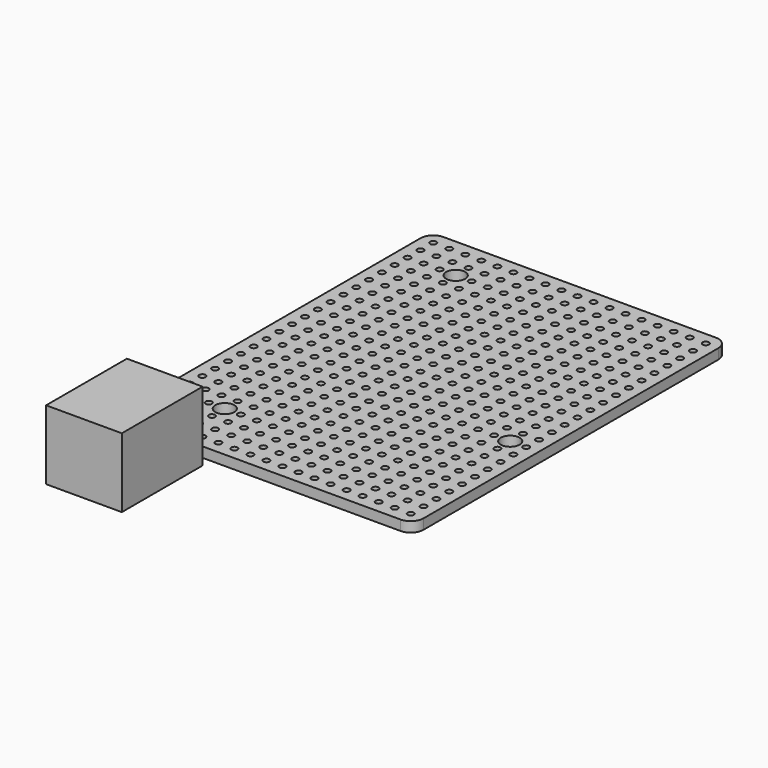
from build123d import *

# Parameters (mm, degrees)
F0_W     = 47.18
F0_H     = 62.42
F0_R     = 0.5
F0_R_2   = 1.5
F1_DEPTH = 1.6
F2_W     = 12
F2_H     = 16
F3_DEPTH = 11
F4_R     = 2


# Not quite as in the source:
# - a feature names something its author has since deleted; it is built from what else it names


with BuildPart() as f1:
    # F0 (on Top) → F1 (new body)
    with BuildSketch(Plane.XY):
        with Locations((-0.5029430622, 18.0375497397)):
            Rectangle(F0_W, F0_H)
        with Locations((-22.0929430622, -11.1724502603)):
            Circle(F0_R, mode=Mode.SUBTRACT)
        with Locations((-19.5529430622, -11.1724502603)):
            Circle(F0_R, mode=Mode.SUBTRACT)
        with Locations((-22.0929430622, -8.6324502603)):
            Circle(F0_R, mode=Mode.SUBTRACT)
        with Locations((-22.0929430622, -6.0924502603)):
            Circle(F0_R, mode=Mode.SUBTRACT)
        with Locations((-19.5529430622, -8.6324502603)):
            Circle(F0_R, mode=Mode.SUBTRACT)
        with Locations((-19.5529430622, -6.0924502603)):
            Circle(F0_R, mode=Mode.SUBTRACT)
        with Locations((-17.0129430622, -11.1724502603)):
            Circle(F0_R, mode=Mode.SUBTRACT)
        with Locations((-14.4729430622, -11.1724502603)):
            Circle(F0_R, mode=Mode.SUBTRACT)
        with Locations((-17.0129430622, -8.6324502603)):
            Circle(F0_R, mode=Mode.SUBTRACT)
        with Locations((-17.0129430622, -6.0924502603)):
            Circle(F0_R, mode=Mode.SUBTRACT)
        with Locations((-14.4729430622, -8.6324502603)):
            Circle(F0_R, mode=Mode.SUBTRACT)
        with Locations((-14.4729430622, -6.0924502603)):
            Circle(F0_R, mode=Mode.SUBTRACT)
        with Locations((-22.0929430622, -3.5524502603)):
            Circle(F0_R, mode=Mode.SUBTRACT)
        with Locations((-19.5529430622, -3.5524502603)):
            Circle(F0_R, mode=Mode.SUBTRACT)
        with Locations((-22.0929430622, -1.0124502603)):
            Circle(F0_R, mode=Mode.SUBTRACT)
        with Locations((-22.0929430622, 1.5275497397)):
            Circle(F0_R, mode=Mode.SUBTRACT)
        with Locations((-19.5529430622, -1.0124502603)):
            Circle(F0_R, mode=Mode.SUBTRACT)
        with Locations((-19.5529430622, 1.5275497397)):
            Circle(F0_R, mode=Mode.SUBTRACT)
        with Locations((-17.0129430622, -3.5524502603)):
            Circle(F0_R, mode=Mode.SUBTRACT)
        with Locations((-14.4729430622, -3.5524502603)):
            Circle(F0_R_2, mode=Mode.SUBTRACT)
        with Locations((-17.0129430622, -1.0124502603)):
            Circle(F0_R, mode=Mode.SUBTRACT)
        with Locations((-17.0129430622, 1.5275497397)):
            Circle(F0_R, mode=Mode.SUBTRACT)
        with Locations((-14.4729430622, -1.0124502603)):
            Circle(F0_R, mode=Mode.SUBTRACT)
        with Locations((-14.4729430622, 1.5275497397)):
            Circle(F0_R, mode=Mode.SUBTRACT)
        with Locations((-11.9329430622, -11.1724502603)):
            Circle(F0_R, mode=Mode.SUBTRACT)
        with Locations((-9.3929430622, -11.1724502603)):
            Circle(F0_R, mode=Mode.SUBTRACT)
        with Locations((-6.8529430622, -11.1724502603)):
            Circle(F0_R, mode=Mode.SUBTRACT)
        with Locations((-11.9329430622, -8.6324502603)):
            Circle(F0_R, mode=Mode.SUBTRACT)
        with Locations((-9.3929430622, -8.6324502603)):
            Circle(F0_R, mode=Mode.SUBTRACT)
        with Locations((-11.9329430622, -6.0924502603)):
            Circle(F0_R, mode=Mode.SUBTRACT)
        with Locations((-9.3929430622, -6.0924502603)):
            Circle(F0_R, mode=Mode.SUBTRACT)
        with Locations((-6.8529430622, -8.6324502603)):
            Circle(F0_R, mode=Mode.SUBTRACT)
        with Locations((-6.8529430622, -6.0924502603)):
            Circle(F0_R, mode=Mode.SUBTRACT)
        with Locations((-4.3129430622, -11.1724502603)):
            Circle(F0_R, mode=Mode.SUBTRACT)
        with Locations((-1.7729430622, -11.1724502603)):
            Circle(F0_R, mode=Mode.SUBTRACT)
        with Locations((-4.3129430622, -8.6324502603)):
            Circle(F0_R, mode=Mode.SUBTRACT)
        with Locations((-4.3129430622, -6.0924502603)):
            Circle(F0_R, mode=Mode.SUBTRACT)
        with Locations((-1.7729430622, -8.6324502603)):
            Circle(F0_R, mode=Mode.SUBTRACT)
        with Locations((-1.7729430622, -6.0924502603)):
            Circle(F0_R, mode=Mode.SUBTRACT)
        with Locations((-11.9329430622, -3.5524502603)):
            Circle(F0_R, mode=Mode.SUBTRACT)
        with Locations((-9.3929430622, -3.5524502603)):
            Circle(F0_R, mode=Mode.SUBTRACT)
        with Locations((-6.8529430622, -3.5524502603)):
            Circle(F0_R, mode=Mode.SUBTRACT)
        with Locations((-11.9329430622, -1.0124502603)):
            Circle(F0_R, mode=Mode.SUBTRACT)
        with Locations((-9.3929430622, -1.0124502603)):
            Circle(F0_R, mode=Mode.SUBTRACT)
        with Locations((-11.9329430622, 1.5275497397)):
            Circle(F0_R, mode=Mode.SUBTRACT)
        with Locations((-9.3929430622, 1.5275497397)):
            Circle(F0_R, mode=Mode.SUBTRACT)
        with Locations((-6.8529430622, -1.0124502603)):
            Circle(F0_R, mode=Mode.SUBTRACT)
        with Locations((-6.8529430622, 1.5275497397)):
            Circle(F0_R, mode=Mode.SUBTRACT)
        with Locations((-4.3129430622, -3.5524502603)):
            Circle(F0_R, mode=Mode.SUBTRACT)
        with Locations((-1.7729430622, -3.5524502603)):
            Circle(F0_R, mode=Mode.SUBTRACT)
        with Locations((-4.3129430622, -1.0124502603)):
            Circle(F0_R, mode=Mode.SUBTRACT)
        with Locations((-4.3129430622, 1.5275497397)):
            Circle(F0_R, mode=Mode.SUBTRACT)
        with Locations((-1.7729430622, -1.0124502603)):
            Circle(F0_R, mode=Mode.SUBTRACT)
        with Locations((-1.7729430622, 1.5275497397)):
            Circle(F0_R, mode=Mode.SUBTRACT)
        with Locations((-22.0929430622, 4.0675497397)):
            Circle(F0_R, mode=Mode.SUBTRACT)
        with Locations((-19.5529430622, 4.0675497397)):
            Circle(F0_R, mode=Mode.SUBTRACT)
        with Locations((-22.0929430622, 6.6075497397)):
            Circle(F0_R, mode=Mode.SUBTRACT)
        with Locations((-22.0929430622, 9.1475497397)):
            Circle(F0_R, mode=Mode.SUBTRACT)
        with Locations((-19.5529430622, 6.6075497397)):
            Circle(F0_R, mode=Mode.SUBTRACT)
        with Locations((-19.5529430622, 9.1475497397)):
            Circle(F0_R, mode=Mode.SUBTRACT)
        with Locations((-17.0129430622, 4.0675497397)):
            Circle(F0_R, mode=Mode.SUBTRACT)
        with Locations((-14.4729430622, 4.0675497397)):
            Circle(F0_R, mode=Mode.SUBTRACT)
        with Locations((-17.0129430622, 6.6075497397)):
            Circle(F0_R, mode=Mode.SUBTRACT)
        with Locations((-17.0129430622, 9.1475497397)):
            Circle(F0_R, mode=Mode.SUBTRACT)
        with Locations((-14.4729430622, 6.6075497397)):
            Circle(F0_R, mode=Mode.SUBTRACT)
        with Locations((-14.4729430622, 9.1475497397)):
            Circle(F0_R, mode=Mode.SUBTRACT)
        with Locations((-22.0929430622, 11.6875497397)):
            Circle(F0_R, mode=Mode.SUBTRACT)
        with Locations((-19.5529430622, 11.6875497397)):
            Circle(F0_R, mode=Mode.SUBTRACT)
        with Locations((-22.0929430622, 14.2275497397)):
            Circle(F0_R, mode=Mode.SUBTRACT)
        with Locations((-22.0929430622, 16.7675497397)):
            Circle(F0_R, mode=Mode.SUBTRACT)
        with Locations((-19.5529430622, 14.2275497397)):
            Circle(F0_R, mode=Mode.SUBTRACT)
        with Locations((-19.5529430622, 16.7675497397)):
            Circle(F0_R, mode=Mode.SUBTRACT)
        with Locations((-17.0129430622, 11.6875497397)):
            Circle(F0_R, mode=Mode.SUBTRACT)
        with Locations((-14.4729430622, 11.6875497397)):
            Circle(F0_R, mode=Mode.SUBTRACT)
        with Locations((-17.0129430622, 14.2275497397)):
            Circle(F0_R, mode=Mode.SUBTRACT)
        with Locations((-17.0129430622, 16.7675497397)):
            Circle(F0_R, mode=Mode.SUBTRACT)
        with Locations((-14.4729430622, 14.2275497397)):
            Circle(F0_R, mode=Mode.SUBTRACT)
        with Locations((-14.4729430622, 16.7675497397)):
            Circle(F0_R, mode=Mode.SUBTRACT)
        with Locations((-11.9329430622, 4.0675497397)):
            Circle(F0_R, mode=Mode.SUBTRACT)
        with Locations((-9.3929430622, 4.0675497397)):
            Circle(F0_R, mode=Mode.SUBTRACT)
        with Locations((-6.8529430622, 4.0675497397)):
            Circle(F0_R, mode=Mode.SUBTRACT)
        with Locations((-11.9329430622, 6.6075497397)):
            Circle(F0_R, mode=Mode.SUBTRACT)
        with Locations((-9.3929430622, 6.6075497397)):
            Circle(F0_R, mode=Mode.SUBTRACT)
        with Locations((-11.9329430622, 9.1475497397)):
            Circle(F0_R, mode=Mode.SUBTRACT)
        with Locations((-9.3929430622, 9.1475497397)):
            Circle(F0_R, mode=Mode.SUBTRACT)
        with Locations((-6.8529430622, 6.6075497397)):
            Circle(F0_R, mode=Mode.SUBTRACT)
        with Locations((-6.8529430622, 9.1475497397)):
            Circle(F0_R, mode=Mode.SUBTRACT)
        with Locations((-4.3129430622, 4.0675497397)):
            Circle(F0_R, mode=Mode.SUBTRACT)
        with Locations((-1.7729430622, 4.0675497397)):
            Circle(F0_R, mode=Mode.SUBTRACT)
        with Locations((-4.3129430622, 6.6075497397)):
            Circle(F0_R, mode=Mode.SUBTRACT)
        with Locations((-4.3129430622, 9.1475497397)):
            Circle(F0_R, mode=Mode.SUBTRACT)
        with Locations((-1.7729430622, 6.6075497397)):
            Circle(F0_R, mode=Mode.SUBTRACT)
        with Locations((-1.7729430622, 9.1475497397)):
            Circle(F0_R, mode=Mode.SUBTRACT)
        with Locations((-11.9329430622, 11.6875497397)):
            Circle(F0_R, mode=Mode.SUBTRACT)
        with Locations((-9.3929430622, 11.6875497397)):
            Circle(F0_R, mode=Mode.SUBTRACT)
        with Locations((-6.8529430622, 11.6875497397)):
            Circle(F0_R, mode=Mode.SUBTRACT)
        with Locations((-11.9329430622, 14.2275497397)):
            Circle(F0_R, mode=Mode.SUBTRACT)
        with Locations((-9.3929430622, 14.2275497397)):
            Circle(F0_R, mode=Mode.SUBTRACT)
        with Locations((-11.9329430622, 16.7675497397)):
            Circle(F0_R, mode=Mode.SUBTRACT)
        with Locations((-9.3929430622, 16.7675497397)):
            Circle(F0_R, mode=Mode.SUBTRACT)
        with Locations((-6.8529430622, 14.2275497397)):
            Circle(F0_R, mode=Mode.SUBTRACT)
        with Locations((-6.8529430622, 16.7675497397)):
            Circle(F0_R, mode=Mode.SUBTRACT)
        with Locations((-4.3129430622, 11.6875497397)):
            Circle(F0_R, mode=Mode.SUBTRACT)
        with Locations((-1.7729430622, 11.6875497397)):
            Circle(F0_R, mode=Mode.SUBTRACT)
        with Locations((-4.3129430622, 14.2275497397)):
            Circle(F0_R, mode=Mode.SUBTRACT)
        with Locations((-4.3129430622, 16.7675497397)):
            Circle(F0_R, mode=Mode.SUBTRACT)
        with Locations((-1.7729430622, 14.2275497397)):
            Circle(F0_R, mode=Mode.SUBTRACT)
        with Locations((-1.7729430622, 16.7675497397)):
            Circle(F0_R, mode=Mode.SUBTRACT)
        with Locations((0.7670569378, -11.1724502603)):
            Circle(F0_R, mode=Mode.SUBTRACT)
        with Locations((3.3070569378, -11.1724502603)):
            Circle(F0_R, mode=Mode.SUBTRACT)
        with Locations((0.7670569378, -8.6324502603)):
            Circle(F0_R, mode=Mode.SUBTRACT)
        with Locations((0.7670569378, -6.0924502603)):
            Circle(F0_R, mode=Mode.SUBTRACT)
        with Locations((3.3070569378, -8.6324502603)):
            Circle(F0_R, mode=Mode.SUBTRACT)
        with Locations((3.3070569378, -6.0924502603)):
            Circle(F0_R, mode=Mode.SUBTRACT)
        with Locations((5.8470569378, -11.1724502603)):
            Circle(F0_R, mode=Mode.SUBTRACT)
        with Locations((8.3870569378, -11.1724502603)):
            Circle(F0_R, mode=Mode.SUBTRACT)
        with Locations((10.9270569378, -11.1724502603)):
            Circle(F0_R, mode=Mode.SUBTRACT)
        with Locations((5.8470569378, -8.6324502603)):
            Circle(F0_R, mode=Mode.SUBTRACT)
        with Locations((5.8470569378, -6.0924502603)):
            Circle(F0_R, mode=Mode.SUBTRACT)
        with Locations((8.3870569378, -8.6324502603)):
            Circle(F0_R, mode=Mode.SUBTRACT)
        with Locations((10.9270569378, -8.6324502603)):
            Circle(F0_R, mode=Mode.SUBTRACT)
        with Locations((8.3870569378, -6.0924502603)):
            Circle(F0_R, mode=Mode.SUBTRACT)
        with Locations((10.9270569378, -6.0924502603)):
            Circle(F0_R, mode=Mode.SUBTRACT)
        with Locations((0.7670569378, -3.5524502603)):
            Circle(F0_R, mode=Mode.SUBTRACT)
        with Locations((3.3070569378, -3.5524502603)):
            Circle(F0_R, mode=Mode.SUBTRACT)
        with Locations((0.7670569378, -1.0124502603)):
            Circle(F0_R, mode=Mode.SUBTRACT)
        with Locations((0.7670569378, 1.5275497397)):
            Circle(F0_R, mode=Mode.SUBTRACT)
        with Locations((3.3070569378, -1.0124502603)):
            Circle(F0_R, mode=Mode.SUBTRACT)
        with Locations((3.3070569378, 1.5275497397)):
            Circle(F0_R, mode=Mode.SUBTRACT)
        with Locations((5.8470569378, -3.5524502603)):
            Circle(F0_R, mode=Mode.SUBTRACT)
        with Locations((8.3870569378, -3.5524502603)):
            Circle(F0_R, mode=Mode.SUBTRACT)
        with Locations((10.9270569378, -3.5524502603)):
            Circle(F0_R, mode=Mode.SUBTRACT)
        with Locations((5.8470569378, -1.0124502603)):
            Circle(F0_R, mode=Mode.SUBTRACT)
        with Locations((5.8470569378, 1.5275497397)):
            Circle(F0_R, mode=Mode.SUBTRACT)
        with Locations((8.3870569378, -1.0124502603)):
            Circle(F0_R, mode=Mode.SUBTRACT)
        with Locations((10.9270569378, -1.0124502603)):
            Circle(F0_R, mode=Mode.SUBTRACT)
        with Locations((8.3870569378, 1.5275497397)):
            Circle(F0_R, mode=Mode.SUBTRACT)
        with Locations((10.9270569378, 1.5275497397)):
            Circle(F0_R, mode=Mode.SUBTRACT)
        with Locations((13.4670569378, -11.1724502603)):
            Circle(F0_R, mode=Mode.SUBTRACT)
        with Locations((16.0070569378, -11.1724502603)):
            Circle(F0_R, mode=Mode.SUBTRACT)
        with Locations((13.4670569378, -8.6324502603)):
            Circle(F0_R, mode=Mode.SUBTRACT)
        with Locations((13.4670569378, -6.0924502603)):
            Circle(F0_R, mode=Mode.SUBTRACT)
        with Locations((16.0070569378, -8.6324502603)):
            Circle(F0_R, mode=Mode.SUBTRACT)
        with Locations((16.0070569378, -6.0924502603)):
            Circle(F0_R, mode=Mode.SUBTRACT)
        with Locations((18.5470569378, -11.1724502603)):
            Circle(F0_R, mode=Mode.SUBTRACT)
        with Locations((21.0870569378, -11.1724502603)):
            Circle(F0_R, mode=Mode.SUBTRACT)
        with Locations((18.5470569378, -8.6324502603)):
            Circle(F0_R, mode=Mode.SUBTRACT)
        with Locations((18.5470569378, -6.0924502603)):
            Circle(F0_R, mode=Mode.SUBTRACT)
        with Locations((21.0870569378, -8.6324502603)):
            Circle(F0_R, mode=Mode.SUBTRACT)
        with Locations((21.0870569378, -6.0924502603)):
            Circle(F0_R, mode=Mode.SUBTRACT)
        with Locations((13.4670569378, -3.5524502603)):
            Circle(F0_R, mode=Mode.SUBTRACT)
        with Locations((16.0070569378, -3.5524502603)):
            Circle(F0_R, mode=Mode.SUBTRACT)
        with Locations((13.4670569378, -1.0124502603)):
            Circle(F0_R, mode=Mode.SUBTRACT)
        with Locations((13.4670569378, 1.5275497397)):
            Circle(F0_R, mode=Mode.SUBTRACT)
        with Locations((16.0070569378, -1.0124502603)):
            Circle(F0_R, mode=Mode.SUBTRACT)
        with Locations((16.0070569378, 1.5275497397)):
            Circle(F0_R, mode=Mode.SUBTRACT)
        with Locations((18.5470569378, -3.5524502603)):
            Circle(F0_R, mode=Mode.SUBTRACT)
        with Locations((21.0870569378, -3.5524502603)):
            Circle(F0_R, mode=Mode.SUBTRACT)
        with Locations((18.5470569378, -1.0124502603)):
            Circle(F0_R, mode=Mode.SUBTRACT)
        with Locations((18.5470569378, 1.5275497397)):
            Circle(F0_R, mode=Mode.SUBTRACT)
        with Locations((21.0870569378, -1.0124502603)):
            Circle(F0_R, mode=Mode.SUBTRACT)
        with Locations((21.0870569378, 1.5275497397)):
            Circle(F0_R, mode=Mode.SUBTRACT)
        with Locations((0.7670569378, 4.0675497397)):
            Circle(F0_R, mode=Mode.SUBTRACT)
        with Locations((3.3070569378, 4.0675497397)):
            Circle(F0_R, mode=Mode.SUBTRACT)
        with Locations((0.7670569378, 6.6075497397)):
            Circle(F0_R, mode=Mode.SUBTRACT)
        with Locations((0.7670569378, 9.1475497397)):
            Circle(F0_R, mode=Mode.SUBTRACT)
        with Locations((3.3070569378, 6.6075497397)):
            Circle(F0_R, mode=Mode.SUBTRACT)
        with Locations((3.3070569378, 9.1475497397)):
            Circle(F0_R, mode=Mode.SUBTRACT)
        with Locations((5.8470569378, 4.0675497397)):
            Circle(F0_R, mode=Mode.SUBTRACT)
        with Locations((8.3870569378, 4.0675497397)):
            Circle(F0_R, mode=Mode.SUBTRACT)
        with Locations((10.9270569378, 4.0675497397)):
            Circle(F0_R, mode=Mode.SUBTRACT)
        with Locations((5.8470569378, 6.6075497397)):
            Circle(F0_R, mode=Mode.SUBTRACT)
        with Locations((5.8470569378, 9.1475497397)):
            Circle(F0_R, mode=Mode.SUBTRACT)
        with Locations((8.3870569378, 6.6075497397)):
            Circle(F0_R, mode=Mode.SUBTRACT)
        with Locations((10.9270569378, 6.6075497397)):
            Circle(F0_R, mode=Mode.SUBTRACT)
        with Locations((8.3870569378, 9.1475497397)):
            Circle(F0_R, mode=Mode.SUBTRACT)
        with Locations((10.9270569378, 9.1475497397)):
            Circle(F0_R, mode=Mode.SUBTRACT)
        with Locations((0.7670569378, 11.6875497397)):
            Circle(F0_R, mode=Mode.SUBTRACT)
        with Locations((3.3070569378, 11.6875497397)):
            Circle(F0_R, mode=Mode.SUBTRACT)
        with Locations((0.7670569378, 14.2275497397)):
            Circle(F0_R, mode=Mode.SUBTRACT)
        with Locations((0.7670569378, 16.7675497397)):
            Circle(F0_R, mode=Mode.SUBTRACT)
        with Locations((3.3070569378, 14.2275497397)):
            Circle(F0_R, mode=Mode.SUBTRACT)
        with Locations((3.3070569378, 16.7675497397)):
            Circle(F0_R, mode=Mode.SUBTRACT)
        with Locations((5.8470569378, 11.6875497397)):
            Circle(F0_R, mode=Mode.SUBTRACT)
        with Locations((8.3870569378, 11.6875497397)):
            Circle(F0_R, mode=Mode.SUBTRACT)
        with Locations((10.9270569378, 11.6875497397)):
            Circle(F0_R, mode=Mode.SUBTRACT)
        with Locations((5.8470569378, 14.2275497397)):
            Circle(F0_R, mode=Mode.SUBTRACT)
        with Locations((5.8470569378, 16.7675497397)):
            Circle(F0_R, mode=Mode.SUBTRACT)
        with Locations((8.3870569378, 14.2275497397)):
            Circle(F0_R, mode=Mode.SUBTRACT)
        with Locations((10.9270569378, 14.2275497397)):
            Circle(F0_R, mode=Mode.SUBTRACT)
        with Locations((8.3870569378, 16.7675497397)):
            Circle(F0_R, mode=Mode.SUBTRACT)
        with Locations((10.9270569378, 16.7675497397)):
            Circle(F0_R, mode=Mode.SUBTRACT)
        with Locations((13.4670569378, 4.0675497397)):
            Circle(F0_R, mode=Mode.SUBTRACT)
        with Locations((16.0070569378, 4.0675497397)):
            Circle(F0_R, mode=Mode.SUBTRACT)
        with Locations((13.4670569378, 6.6075497397)):
            Circle(F0_R, mode=Mode.SUBTRACT)
        with Locations((13.4670569378, 9.1475497397)):
            Circle(F0_R, mode=Mode.SUBTRACT)
        with Locations((16.0070569378, 6.6075497397)):
            Circle(F0_R, mode=Mode.SUBTRACT)
        with Locations((16.0070569378, 9.1475497397)):
            Circle(F0_R, mode=Mode.SUBTRACT)
        with Locations((18.5470569378, 4.0675497397)):
            Circle(F0_R, mode=Mode.SUBTRACT)
        with Locations((21.0870569378, 4.0675497397)):
            Circle(F0_R, mode=Mode.SUBTRACT)
        with Locations((18.5470569378, 6.6075497397)):
            Circle(F0_R, mode=Mode.SUBTRACT)
        with Locations((18.5470569378, 9.1475497397)):
            Circle(F0_R, mode=Mode.SUBTRACT)
        with Locations((21.0870569378, 6.6075497397)):
            Circle(F0_R, mode=Mode.SUBTRACT)
        with Locations((21.0870569378, 9.1475497397)):
            Circle(F0_R, mode=Mode.SUBTRACT)
        with Locations((13.4670569378, 11.6875497397)):
            Circle(F0_R, mode=Mode.SUBTRACT)
        with Locations((16.0070569378, 11.6875497397)):
            Circle(F0_R, mode=Mode.SUBTRACT)
        with Locations((13.4670569378, 14.2275497397)):
            Circle(F0_R, mode=Mode.SUBTRACT)
        with Locations((13.4670569378, 16.7675497397)):
            Circle(F0_R, mode=Mode.SUBTRACT)
        with Locations((16.0070569378, 14.2275497397)):
            Circle(F0_R, mode=Mode.SUBTRACT)
        with Locations((16.0070569378, 16.7675497397)):
            Circle(F0_R, mode=Mode.SUBTRACT)
        with Locations((18.5470569378, 11.6875497397)):
            Circle(F0_R_2, mode=Mode.SUBTRACT)
        with Locations((21.0870569378, 11.6875497397)):
            Circle(F0_R, mode=Mode.SUBTRACT)
        with Locations((18.5470569378, 14.2275497397)):
            Circle(F0_R, mode=Mode.SUBTRACT)
        with Locations((18.5470569378, 16.7675497397)):
            Circle(F0_R, mode=Mode.SUBTRACT)
        with Locations((21.0870569378, 14.2275497397)):
            Circle(F0_R, mode=Mode.SUBTRACT)
        with Locations((21.0870569378, 16.7675497397)):
            Circle(F0_R, mode=Mode.SUBTRACT)
        with Locations((-22.0929430622, 19.3075497397)):
            Circle(F0_R, mode=Mode.SUBTRACT)
        with Locations((-22.0929430622, 21.8475497397)):
            Circle(F0_R, mode=Mode.SUBTRACT)
        with Locations((-19.5529430622, 19.3075497397)):
            Circle(F0_R, mode=Mode.SUBTRACT)
        with Locations((-19.5529430622, 21.8475497397)):
            Circle(F0_R, mode=Mode.SUBTRACT)
        with Locations((-22.0929430622, 24.3875497397)):
            Circle(F0_R, mode=Mode.SUBTRACT)
        with Locations((-19.5529430622, 24.3875497397)):
            Circle(F0_R, mode=Mode.SUBTRACT)
        with Locations((-17.0129430622, 19.3075497397)):
            Circle(F0_R, mode=Mode.SUBTRACT)
        with Locations((-17.0129430622, 21.8475497397)):
            Circle(F0_R, mode=Mode.SUBTRACT)
        with Locations((-14.4729430622, 19.3075497397)):
            Circle(F0_R, mode=Mode.SUBTRACT)
        with Locations((-14.4729430622, 21.8475497397)):
            Circle(F0_R, mode=Mode.SUBTRACT)
        with Locations((-17.0129430622, 24.3875497397)):
            Circle(F0_R, mode=Mode.SUBTRACT)
        with Locations((-14.4729430622, 24.3875497397)):
            Circle(F0_R, mode=Mode.SUBTRACT)
        with Locations((-22.0929430622, 26.9275497397)):
            Circle(F0_R, mode=Mode.SUBTRACT)
        with Locations((-22.0929430622, 29.4675497397)):
            Circle(F0_R, mode=Mode.SUBTRACT)
        with Locations((-19.5529430622, 26.9275497397)):
            Circle(F0_R, mode=Mode.SUBTRACT)
        with Locations((-19.5529430622, 29.4675497397)):
            Circle(F0_R, mode=Mode.SUBTRACT)
        with Locations((-22.0929430622, 32.0075497397)):
            Circle(F0_R, mode=Mode.SUBTRACT)
        with Locations((-19.5529430622, 32.0075497397)):
            Circle(F0_R, mode=Mode.SUBTRACT)
        with Locations((-17.0129430622, 26.9275497397)):
            Circle(F0_R, mode=Mode.SUBTRACT)
        with Locations((-17.0129430622, 29.4675497397)):
            Circle(F0_R, mode=Mode.SUBTRACT)
        with Locations((-14.4729430622, 26.9275497397)):
            Circle(F0_R, mode=Mode.SUBTRACT)
        with Locations((-14.4729430622, 29.4675497397)):
            Circle(F0_R, mode=Mode.SUBTRACT)
        with Locations((-17.0129430622, 32.0075497397)):
            Circle(F0_R, mode=Mode.SUBTRACT)
        with Locations((-14.4729430622, 32.0075497397)):
            Circle(F0_R, mode=Mode.SUBTRACT)
        with Locations((-11.9329430622, 19.3075497397)):
            Circle(F0_R, mode=Mode.SUBTRACT)
        with Locations((-9.3929430622, 19.3075497397)):
            Circle(F0_R, mode=Mode.SUBTRACT)
        with Locations((-11.9329430622, 21.8475497397)):
            Circle(F0_R, mode=Mode.SUBTRACT)
        with Locations((-9.3929430622, 21.8475497397)):
            Circle(F0_R, mode=Mode.SUBTRACT)
        with Locations((-6.8529430622, 19.3075497397)):
            Circle(F0_R, mode=Mode.SUBTRACT)
        with Locations((-6.8529430622, 21.8475497397)):
            Circle(F0_R, mode=Mode.SUBTRACT)
        with Locations((-11.9329430622, 24.3875497397)):
            Circle(F0_R, mode=Mode.SUBTRACT)
        with Locations((-9.3929430622, 24.3875497397)):
            Circle(F0_R, mode=Mode.SUBTRACT)
        with Locations((-6.8529430622, 24.3875497397)):
            Circle(F0_R, mode=Mode.SUBTRACT)
        with Locations((-4.3129430622, 19.3075497397)):
            Circle(F0_R, mode=Mode.SUBTRACT)
        with Locations((-4.3129430622, 21.8475497397)):
            Circle(F0_R, mode=Mode.SUBTRACT)
        with Locations((-1.7729430622, 19.3075497397)):
            Circle(F0_R, mode=Mode.SUBTRACT)
        with Locations((-1.7729430622, 21.8475497397)):
            Circle(F0_R, mode=Mode.SUBTRACT)
        with Locations((-4.3129430622, 24.3875497397)):
            Circle(F0_R, mode=Mode.SUBTRACT)
        with Locations((-1.7729430622, 24.3875497397)):
            Circle(F0_R, mode=Mode.SUBTRACT)
        with Locations((-11.9329430622, 26.9275497397)):
            Circle(F0_R, mode=Mode.SUBTRACT)
        with Locations((-9.3929430622, 26.9275497397)):
            Circle(F0_R, mode=Mode.SUBTRACT)
        with Locations((-11.9329430622, 29.4675497397)):
            Circle(F0_R, mode=Mode.SUBTRACT)
        with Locations((-9.3929430622, 29.4675497397)):
            Circle(F0_R, mode=Mode.SUBTRACT)
        with Locations((-6.8529430622, 26.9275497397)):
            Circle(F0_R, mode=Mode.SUBTRACT)
        with Locations((-6.8529430622, 29.4675497397)):
            Circle(F0_R, mode=Mode.SUBTRACT)
        with Locations((-11.9329430622, 32.0075497397)):
            Circle(F0_R, mode=Mode.SUBTRACT)
        with Locations((-9.3929430622, 32.0075497397)):
            Circle(F0_R, mode=Mode.SUBTRACT)
        with Locations((-6.8529430622, 32.0075497397)):
            Circle(F0_R, mode=Mode.SUBTRACT)
        with Locations((-4.3129430622, 26.9275497397)):
            Circle(F0_R, mode=Mode.SUBTRACT)
        with Locations((-4.3129430622, 29.4675497397)):
            Circle(F0_R, mode=Mode.SUBTRACT)
        with Locations((-1.7729430622, 26.9275497397)):
            Circle(F0_R, mode=Mode.SUBTRACT)
        with Locations((-1.7729430622, 29.4675497397)):
            Circle(F0_R, mode=Mode.SUBTRACT)
        with Locations((-4.3129430622, 32.0075497397)):
            Circle(F0_R, mode=Mode.SUBTRACT)
        with Locations((-1.7729430622, 32.0075497397)):
            Circle(F0_R, mode=Mode.SUBTRACT)
        with Locations((-22.0929430622, 34.5475497397)):
            Circle(F0_R, mode=Mode.SUBTRACT)
        with Locations((-22.0929430622, 37.0875497397)):
            Circle(F0_R, mode=Mode.SUBTRACT)
        with Locations((-19.5529430622, 34.5475497397)):
            Circle(F0_R, mode=Mode.SUBTRACT)
        with Locations((-19.5529430622, 37.0875497397)):
            Circle(F0_R, mode=Mode.SUBTRACT)
        with Locations((-22.0929430622, 39.6275497397)):
            Circle(F0_R, mode=Mode.SUBTRACT)
        with Locations((-19.5529430622, 39.6275497397)):
            Circle(F0_R, mode=Mode.SUBTRACT)
        with Locations((-17.0129430622, 34.5475497397)):
            Circle(F0_R, mode=Mode.SUBTRACT)
        with Locations((-17.0129430622, 37.0875497397)):
            Circle(F0_R, mode=Mode.SUBTRACT)
        with Locations((-14.4729430622, 34.5475497397)):
            Circle(F0_R, mode=Mode.SUBTRACT)
        with Locations((-14.4729430622, 37.0875497397)):
            Circle(F0_R, mode=Mode.SUBTRACT)
        with Locations((-17.0129430622, 39.6275497397)):
            Circle(F0_R, mode=Mode.SUBTRACT)
        with Locations((-14.4729430622, 39.6275497397)):
            Circle(F0_R, mode=Mode.SUBTRACT)
        with Locations((-22.0929430622, 42.1675497397)):
            Circle(F0_R, mode=Mode.SUBTRACT)
        with Locations((-22.0929430622, 44.7075497397)):
            Circle(F0_R, mode=Mode.SUBTRACT)
        with Locations((-19.5529430622, 42.1675497397)):
            Circle(F0_R, mode=Mode.SUBTRACT)
        with Locations((-19.5529430622, 44.7075497397)):
            Circle(F0_R, mode=Mode.SUBTRACT)
        with Locations((-22.0929430622, 47.2475497397)):
            Circle(F0_R, mode=Mode.SUBTRACT)
        with Locations((-19.5529430622, 47.2475497397)):
            Circle(F0_R, mode=Mode.SUBTRACT)
        with Locations((-17.0129430622, 42.1675497397)):
            Circle(F0_R, mode=Mode.SUBTRACT)
        with Locations((-17.0129430622, 44.7075497397)):
            Circle(F0_R, mode=Mode.SUBTRACT)
        with Locations((-14.4729430622, 42.1675497397)):
            Circle(F0_R_2, mode=Mode.SUBTRACT)
        with Locations((-14.4729430622, 44.7075497397)):
            Circle(F0_R, mode=Mode.SUBTRACT)
        with Locations((-17.0129430622, 47.2475497397)):
            Circle(F0_R, mode=Mode.SUBTRACT)
        with Locations((-14.4729430622, 47.2475497397)):
            Circle(F0_R, mode=Mode.SUBTRACT)
        with Locations((-11.9329430622, 34.5475497397)):
            Circle(F0_R, mode=Mode.SUBTRACT)
        with Locations((-9.3929430622, 34.5475497397)):
            Circle(F0_R, mode=Mode.SUBTRACT)
        with Locations((-11.9329430622, 37.0875497397)):
            Circle(F0_R, mode=Mode.SUBTRACT)
        with Locations((-9.3929430622, 37.0875497397)):
            Circle(F0_R, mode=Mode.SUBTRACT)
        with Locations((-6.8529430622, 34.5475497397)):
            Circle(F0_R, mode=Mode.SUBTRACT)
        with Locations((-6.8529430622, 37.0875497397)):
            Circle(F0_R, mode=Mode.SUBTRACT)
        with Locations((-11.9329430622, 39.6275497397)):
            Circle(F0_R, mode=Mode.SUBTRACT)
        with Locations((-9.3929430622, 39.6275497397)):
            Circle(F0_R, mode=Mode.SUBTRACT)
        with Locations((-6.8529430622, 39.6275497397)):
            Circle(F0_R, mode=Mode.SUBTRACT)
        with Locations((-4.3129430622, 34.5475497397)):
            Circle(F0_R, mode=Mode.SUBTRACT)
        with Locations((-4.3129430622, 37.0875497397)):
            Circle(F0_R, mode=Mode.SUBTRACT)
        with Locations((-1.7729430622, 34.5475497397)):
            Circle(F0_R, mode=Mode.SUBTRACT)
        with Locations((-1.7729430622, 37.0875497397)):
            Circle(F0_R, mode=Mode.SUBTRACT)
        with Locations((-4.3129430622, 39.6275497397)):
            Circle(F0_R, mode=Mode.SUBTRACT)
        with Locations((-1.7729430622, 39.6275497397)):
            Circle(F0_R, mode=Mode.SUBTRACT)
        with Locations((-11.9329430622, 42.1675497397)):
            Circle(F0_R, mode=Mode.SUBTRACT)
        with Locations((-9.3929430622, 42.1675497397)):
            Circle(F0_R, mode=Mode.SUBTRACT)
        with Locations((-11.9329430622, 44.7075497397)):
            Circle(F0_R, mode=Mode.SUBTRACT)
        with Locations((-9.3929430622, 44.7075497397)):
            Circle(F0_R, mode=Mode.SUBTRACT)
        with Locations((-6.8529430622, 42.1675497397)):
            Circle(F0_R, mode=Mode.SUBTRACT)
        with Locations((-6.8529430622, 44.7075497397)):
            Circle(F0_R, mode=Mode.SUBTRACT)
        with Locations((-11.9329430622, 47.2475497397)):
            Circle(F0_R, mode=Mode.SUBTRACT)
        with Locations((-9.3929430622, 47.2475497397)):
            Circle(F0_R, mode=Mode.SUBTRACT)
        with Locations((-6.8529430622, 47.2475497397)):
            Circle(F0_R, mode=Mode.SUBTRACT)
        with Locations((-4.3129430622, 42.1675497397)):
            Circle(F0_R, mode=Mode.SUBTRACT)
        with Locations((-4.3129430622, 44.7075497397)):
            Circle(F0_R, mode=Mode.SUBTRACT)
        with Locations((-1.7729430622, 42.1675497397)):
            Circle(F0_R, mode=Mode.SUBTRACT)
        with Locations((-1.7729430622, 44.7075497397)):
            Circle(F0_R, mode=Mode.SUBTRACT)
        with Locations((-4.3129430622, 47.2475497397)):
            Circle(F0_R, mode=Mode.SUBTRACT)
        with Locations((-1.7729430622, 47.2475497397)):
            Circle(F0_R, mode=Mode.SUBTRACT)
        with Locations((0.7670569378, 19.3075497397)):
            Circle(F0_R, mode=Mode.SUBTRACT)
        with Locations((0.7670569378, 21.8475497397)):
            Circle(F0_R, mode=Mode.SUBTRACT)
        with Locations((3.3070569378, 19.3075497397)):
            Circle(F0_R, mode=Mode.SUBTRACT)
        with Locations((3.3070569378, 21.8475497397)):
            Circle(F0_R, mode=Mode.SUBTRACT)
        with Locations((0.7670569378, 24.3875497397)):
            Circle(F0_R, mode=Mode.SUBTRACT)
        with Locations((3.3070569378, 24.3875497397)):
            Circle(F0_R, mode=Mode.SUBTRACT)
        with Locations((5.8470569378, 19.3075497397)):
            Circle(F0_R, mode=Mode.SUBTRACT)
        with Locations((5.8470569378, 21.8475497397)):
            Circle(F0_R, mode=Mode.SUBTRACT)
        with Locations((8.3870569378, 19.3075497397)):
            Circle(F0_R, mode=Mode.SUBTRACT)
        with Locations((10.9270569378, 19.3075497397)):
            Circle(F0_R, mode=Mode.SUBTRACT)
        with Locations((8.3870569378, 21.8475497397)):
            Circle(F0_R, mode=Mode.SUBTRACT)
        with Locations((10.9270569378, 21.8475497397)):
            Circle(F0_R, mode=Mode.SUBTRACT)
        with Locations((5.8470569378, 24.3875497397)):
            Circle(F0_R, mode=Mode.SUBTRACT)
        with Locations((8.3870569378, 24.3875497397)):
            Circle(F0_R, mode=Mode.SUBTRACT)
        with Locations((10.9270569378, 24.3875497397)):
            Circle(F0_R, mode=Mode.SUBTRACT)
        with Locations((0.7670569378, 26.9275497397)):
            Circle(F0_R, mode=Mode.SUBTRACT)
        with Locations((0.7670569378, 29.4675497397)):
            Circle(F0_R, mode=Mode.SUBTRACT)
        with Locations((3.3070569378, 26.9275497397)):
            Circle(F0_R, mode=Mode.SUBTRACT)
        with Locations((3.3070569378, 29.4675497397)):
            Circle(F0_R, mode=Mode.SUBTRACT)
        with Locations((0.7670569378, 32.0075497397)):
            Circle(F0_R, mode=Mode.SUBTRACT)
        with Locations((3.3070569378, 32.0075497397)):
            Circle(F0_R, mode=Mode.SUBTRACT)
        with Locations((5.8470569378, 26.9275497397)):
            Circle(F0_R, mode=Mode.SUBTRACT)
        with Locations((5.8470569378, 29.4675497397)):
            Circle(F0_R, mode=Mode.SUBTRACT)
        with Locations((8.3870569378, 26.9275497397)):
            Circle(F0_R, mode=Mode.SUBTRACT)
        with Locations((10.9270569378, 26.9275497397)):
            Circle(F0_R, mode=Mode.SUBTRACT)
        with Locations((8.3870569378, 29.4675497397)):
            Circle(F0_R, mode=Mode.SUBTRACT)
        with Locations((10.9270569378, 29.4675497397)):
            Circle(F0_R, mode=Mode.SUBTRACT)
        with Locations((5.8470569378, 32.0075497397)):
            Circle(F0_R, mode=Mode.SUBTRACT)
        with Locations((8.3870569378, 32.0075497397)):
            Circle(F0_R, mode=Mode.SUBTRACT)
        with Locations((10.9270569378, 32.0075497397)):
            Circle(F0_R, mode=Mode.SUBTRACT)
        with Locations((13.4670569378, 19.3075497397)):
            Circle(F0_R, mode=Mode.SUBTRACT)
        with Locations((13.4670569378, 21.8475497397)):
            Circle(F0_R, mode=Mode.SUBTRACT)
        with Locations((16.0070569378, 19.3075497397)):
            Circle(F0_R, mode=Mode.SUBTRACT)
        with Locations((16.0070569378, 21.8475497397)):
            Circle(F0_R, mode=Mode.SUBTRACT)
        with Locations((13.4670569378, 24.3875497397)):
            Circle(F0_R, mode=Mode.SUBTRACT)
        with Locations((16.0070569378, 24.3875497397)):
            Circle(F0_R, mode=Mode.SUBTRACT)
        with Locations((18.5470569378, 19.3075497397)):
            Circle(F0_R, mode=Mode.SUBTRACT)
        with Locations((18.5470569378, 21.8475497397)):
            Circle(F0_R, mode=Mode.SUBTRACT)
        with Locations((21.0870569378, 19.3075497397)):
            Circle(F0_R, mode=Mode.SUBTRACT)
        with Locations((21.0870569378, 21.8475497397)):
            Circle(F0_R, mode=Mode.SUBTRACT)
        with Locations((18.5470569378, 24.3875497397)):
            Circle(F0_R, mode=Mode.SUBTRACT)
        with Locations((21.0870569378, 24.3875497397)):
            Circle(F0_R, mode=Mode.SUBTRACT)
        with Locations((13.4670569378, 26.9275497397)):
            Circle(F0_R, mode=Mode.SUBTRACT)
        with Locations((13.4670569378, 29.4675497397)):
            Circle(F0_R, mode=Mode.SUBTRACT)
        with Locations((16.0070569378, 26.9275497397)):
            Circle(F0_R, mode=Mode.SUBTRACT)
        with Locations((16.0070569378, 29.4675497397)):
            Circle(F0_R, mode=Mode.SUBTRACT)
        with Locations((13.4670569378, 32.0075497397)):
            Circle(F0_R, mode=Mode.SUBTRACT)
        with Locations((16.0070569378, 32.0075497397)):
            Circle(F0_R, mode=Mode.SUBTRACT)
        with Locations((18.5470569378, 26.9275497397)):
            Circle(F0_R, mode=Mode.SUBTRACT)
        with Locations((18.5470569378, 29.4675497397)):
            Circle(F0_R, mode=Mode.SUBTRACT)
        with Locations((21.0870569378, 26.9275497397)):
            Circle(F0_R, mode=Mode.SUBTRACT)
        with Locations((21.0870569378, 29.4675497397)):
            Circle(F0_R, mode=Mode.SUBTRACT)
        with Locations((18.5470569378, 32.0075497397)):
            Circle(F0_R, mode=Mode.SUBTRACT)
        with Locations((21.0870569378, 32.0075497397)):
            Circle(F0_R, mode=Mode.SUBTRACT)
        with Locations((0.7670569378, 34.5475497397)):
            Circle(F0_R, mode=Mode.SUBTRACT)
        with Locations((0.7670569378, 37.0875497397)):
            Circle(F0_R, mode=Mode.SUBTRACT)
        with Locations((3.3070569378, 34.5475497397)):
            Circle(F0_R, mode=Mode.SUBTRACT)
        with Locations((3.3070569378, 37.0875497397)):
            Circle(F0_R, mode=Mode.SUBTRACT)
        with Locations((0.7670569378, 39.6275497397)):
            Circle(F0_R, mode=Mode.SUBTRACT)
        with Locations((3.3070569378, 39.6275497397)):
            Circle(F0_R, mode=Mode.SUBTRACT)
        with Locations((5.8470569378, 34.5475497397)):
            Circle(F0_R, mode=Mode.SUBTRACT)
        with Locations((5.8470569378, 37.0875497397)):
            Circle(F0_R, mode=Mode.SUBTRACT)
        with Locations((8.3870569378, 34.5475497397)):
            Circle(F0_R, mode=Mode.SUBTRACT)
        with Locations((10.9270569378, 34.5475497397)):
            Circle(F0_R, mode=Mode.SUBTRACT)
        with Locations((8.3870569378, 37.0875497397)):
            Circle(F0_R, mode=Mode.SUBTRACT)
        with Locations((10.9270569378, 37.0875497397)):
            Circle(F0_R, mode=Mode.SUBTRACT)
        with Locations((5.8470569378, 39.6275497397)):
            Circle(F0_R, mode=Mode.SUBTRACT)
        with Locations((8.3870569378, 39.6275497397)):
            Circle(F0_R, mode=Mode.SUBTRACT)
        with Locations((10.9270569378, 39.6275497397)):
            Circle(F0_R, mode=Mode.SUBTRACT)
        with Locations((0.7670569378, 42.1675497397)):
            Circle(F0_R, mode=Mode.SUBTRACT)
        with Locations((0.7670569378, 44.7075497397)):
            Circle(F0_R, mode=Mode.SUBTRACT)
        with Locations((3.3070569378, 42.1675497397)):
            Circle(F0_R, mode=Mode.SUBTRACT)
        with Locations((3.3070569378, 44.7075497397)):
            Circle(F0_R, mode=Mode.SUBTRACT)
        with Locations((0.7670569378, 47.2475497397)):
            Circle(F0_R, mode=Mode.SUBTRACT)
        with Locations((3.3070569378, 47.2475497397)):
            Circle(F0_R, mode=Mode.SUBTRACT)
        with Locations((5.8470569378, 42.1675497397)):
            Circle(F0_R, mode=Mode.SUBTRACT)
        with Locations((5.8470569378, 44.7075497397)):
            Circle(F0_R, mode=Mode.SUBTRACT)
        with Locations((8.3870569378, 42.1675497397)):
            Circle(F0_R, mode=Mode.SUBTRACT)
        with Locations((10.9270569378, 42.1675497397)):
            Circle(F0_R, mode=Mode.SUBTRACT)
        with Locations((8.3870569378, 44.7075497397)):
            Circle(F0_R, mode=Mode.SUBTRACT)
        with Locations((10.9270569378, 44.7075497397)):
            Circle(F0_R, mode=Mode.SUBTRACT)
        with Locations((5.8470569378, 47.2475497397)):
            Circle(F0_R, mode=Mode.SUBTRACT)
        with Locations((8.3870569378, 47.2475497397)):
            Circle(F0_R, mode=Mode.SUBTRACT)
        with Locations((10.9270569378, 47.2475497397)):
            Circle(F0_R, mode=Mode.SUBTRACT)
        with Locations((13.4670569378, 34.5475497397)):
            Circle(F0_R, mode=Mode.SUBTRACT)
        with Locations((13.4670569378, 37.0875497397)):
            Circle(F0_R, mode=Mode.SUBTRACT)
        with Locations((16.0070569378, 34.5475497397)):
            Circle(F0_R, mode=Mode.SUBTRACT)
        with Locations((16.0070569378, 37.0875497397)):
            Circle(F0_R, mode=Mode.SUBTRACT)
        with Locations((13.4670569378, 39.6275497397)):
            Circle(F0_R, mode=Mode.SUBTRACT)
        with Locations((16.0070569378, 39.6275497397)):
            Circle(F0_R, mode=Mode.SUBTRACT)
        with Locations((18.5470569378, 34.5475497397)):
            Circle(F0_R, mode=Mode.SUBTRACT)
        with Locations((18.5470569378, 37.0875497397)):
            Circle(F0_R, mode=Mode.SUBTRACT)
        with Locations((21.0870569378, 34.5475497397)):
            Circle(F0_R, mode=Mode.SUBTRACT)
        with Locations((21.0870569378, 37.0875497397)):
            Circle(F0_R, mode=Mode.SUBTRACT)
        with Locations((18.5470569378, 39.6275497397)):
            Circle(F0_R, mode=Mode.SUBTRACT)
        with Locations((21.0870569378, 39.6275497397)):
            Circle(F0_R, mode=Mode.SUBTRACT)
        with Locations((13.4670569378, 42.1675497397)):
            Circle(F0_R, mode=Mode.SUBTRACT)
        with Locations((13.4670569378, 44.7075497397)):
            Circle(F0_R, mode=Mode.SUBTRACT)
        with Locations((16.0070569378, 42.1675497397)):
            Circle(F0_R, mode=Mode.SUBTRACT)
        with Locations((16.0070569378, 44.7075497397)):
            Circle(F0_R, mode=Mode.SUBTRACT)
        with Locations((13.4670569378, 47.2475497397)):
            Circle(F0_R, mode=Mode.SUBTRACT)
        with Locations((16.0070569378, 47.2475497397)):
            Circle(F0_R, mode=Mode.SUBTRACT)
        with Locations((18.5470569378, 42.1675497397)):
            Circle(F0_R, mode=Mode.SUBTRACT)
        with Locations((18.5470569378, 44.7075497397)):
            Circle(F0_R, mode=Mode.SUBTRACT)
        with Locations((21.0870569378, 42.1675497397)):
            Circle(F0_R, mode=Mode.SUBTRACT)
        with Locations((21.0870569378, 44.7075497397)):
            Circle(F0_R, mode=Mode.SUBTRACT)
        with Locations((18.5470569378, 47.2475497397)):
            Circle(F0_R, mode=Mode.SUBTRACT)
        with Locations((21.0870569378, 47.2475497397)):
            Circle(F0_R, mode=Mode.SUBTRACT)
    extrude(amount=F1_DEPTH)

    # F4
    f4_edges = [f1.edges().sort_by_distance(p)[0] for p in [
        (-24.092943, -13.17245, 0.8),
        (-24.092943, 49.24755, 0.8),
        (23.087057, 49.24755, 0.8),
        (23.087057, -13.17245, 0.8),
    ]]
    fillet(f4_edges, radius=F4_R)


with BuildPart() as f3:
    # F2 (on face) → F3 (new body)
    with BuildSketch(Plane.XY.offset(1.6)):
        with Locations((-13.0929430622, -25.1724502603)):
            Rectangle(F2_W, F2_H)
    extrude(amount=F3_DEPTH)


solid = Compound([f1.part, f3.part])
